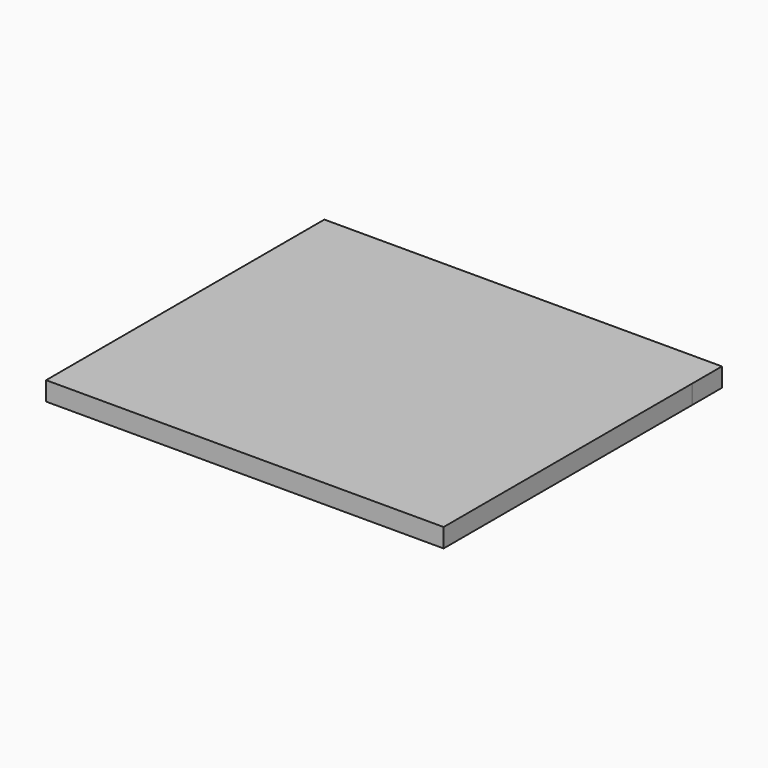
from build123d import *

# Parameters (mm, degrees)
F1_DEPTH = 19
F2_DEPTH = 548
F3_DEPTH = 548


# Not quite as in the source:
# - an extrude ends at something that could not be found from the text; its depth is read off the source's solid


with BuildPart() as f1:
    # F0 (on Top) → F1 (new body)
    with BuildSketch(Plane.XY):
        with BuildLine():
            add(Edge.make_bspline(
                [(-200, -132.6209452411), (-200, -154.8058367287), (-187.1411707237, -172.3375741418), (-168.017625666, -187.1492117643), (-133.0151869916, -187.1492117643)],
                knots=[0, 0, 0, 0, 0.4562793143, 1, 1, 1, 1], degree=3))
            Line((-200, -132.6209452411), (-200, -187.1492117643))
            Line((-200, -187.1492117643), (-133.0151869916, -187.1492117643))
        make_face()
        with BuildLine():
            Line((200, -187.1492117643), (200, -133.3316862583))
            add(Edge.make_bspline(
                [(200, -133.3316862583), (196.8726040376, -145.854416396), (194.7195639705, -177.063078406), (166.3433221251, -183.7126432901), (157.4708074331, -187.1492117643)],
                knots=[0, 0, 0, 0, 0.5227747717, 1, 1, 1, 1], degree=3))
            Line((157.4708074331, -187.1492117643), (200, -187.1492117643))
        make_face()
        with BuildLine():
            add(Edge.make_bspline(
                [(200, 125.7612258196), (200.0567834577, 125.2951155246), (200.0345329904, 125.1404634173), (200, 124.9924004078)],
                knots=[0.9249687191, 0.9249687191, 0.9249687191, 0.9249687191, 1, 1, 1, 1], degree=3))
            Line((200, 125.7612258196), (200, 124.9924004078))
        make_face()
        with BuildLine():
            add(Edge.make_bspline(
                [(159.7772687674, 162.8507882357), (169.0774328446, 160.2876502356), (193.3291623418, 156.440564551), (199.6711808851, 128.4603565342), (200, 125.7612258196)],
                knots=[0, 0, 0, 0, 0.4904809229, 0.9249687191, 0.9249687191, 0.9249687191, 0.9249687191], degree=3))
            Line((159.7772687674, 162.8507882357), (-153.6801122603, 162.8507882357))
            add(Edge.make_bspline(
                [(-200, 104.9124646716), (-200, 131.7387589341), (-185.8746875729, 148.9797410683), (-171.5849838132, 162.8507882357), (-153.6801122603, 162.8507882357)],
                knots=[0, 0, 0, 0, 0.5414752597, 1, 1, 1, 1], degree=3))
            Line((-200, 104.9124646716), (-200, -132.6209452411))
            add(Edge.make_bspline(
                [(-200, -132.6209452411), (-200, -154.8058367287), (-187.1411707237, -172.3375741418), (-168.017625666, -187.1492117643), (-133.0151869916, -187.1492117643)],
                knots=[0, 0, 0, 0, 0.4562793143, 1, 1, 1, 1], degree=3))
            Line((-133.0151869916, -187.1492117643), (157.4708074331, -187.1492117643))
            add(Edge.make_bspline(
                [(200, -133.3316862583), (196.8726040376, -145.854416396), (194.7195639705, -177.063078406), (166.3433221251, -183.7126432901), (157.4708074331, -187.1492117643)],
                knots=[0, 0, 0, 0, 0.5227747717, 1, 1, 1, 1], degree=3))
            Line((200, -133.3316862583), (200, 124.9924004078))
            Line((200, 124.9924004078), (200, 125.7612258196))
        make_face()
        with BuildLine():
            add(Edge.make_bspline(
                [(-200, 104.9124646716), (-200, 131.7387589341), (-185.8746875729, 148.9797410683), (-171.5849838132, 162.8507882357), (-153.6801122603, 162.8507882357)],
                knots=[0, 0, 0, 0, 0.5414752597, 1, 1, 1, 1], degree=3))
            Line((-153.6801122603, 162.8507882357), (-200, 162.8507882357))
            Line((-200, 162.8507882357), (-200, 104.9124646716))
        make_face()
        with BuildLine():
            Line((200, 125.7612258196), (200, 162.8507882357))
            Line((200, 162.8507882357), (159.7772687674, 162.8507882357))
            add(Edge.make_bspline(
                [(159.7772687674, 162.8507882357), (169.0774328446, 160.2876502356), (193.3291623418, 156.440564551), (199.6711808851, 128.4603565342), (200, 125.7612258196)],
                knots=[0, 0, 0, 0, 0.4904809229, 0.9249687191, 0.9249687191, 0.9249687191, 0.9249687191], degree=3))
        make_face()
    extrude(amount=F1_DEPTH)

    # F0 (on Top) → F2 (cut, through all)
    with BuildSketch(Plane.XY):
        with BuildLine():
            add(Edge.make_bspline(
                [(-200, -132.6209452411), (-200, -154.8058367287), (-187.1411707237, -172.3375741418), (-168.017625666, -187.1492117643), (-133.0151869916, -187.1492117643)],
                knots=[0, 0, 0, 0, 0.4562793143, 1, 1, 1, 1], degree=3))
            Line((-200, -132.6209452411), (-200, -187.1492117643))
            Line((-200, -187.1492117643), (-133.0151869916, -187.1492117643))
        make_face()
    extrude(amount=-F2_DEPTH, mode=Mode.SUBTRACT)

    # F0 (on Top) → F3 (cut, through all)
    with BuildSketch(Plane.XY):
        with BuildLine():
            add(Edge.make_bspline(
                [(-200, 104.9124646716), (-200, 131.7387589341), (-185.8746875729, 148.9797410683), (-171.5849838132, 162.8507882357), (-153.6801122603, 162.8507882357)],
                knots=[0, 0, 0, 0, 0.5414752597, 1, 1, 1, 1], degree=3))
            Line((-153.6801122603, 162.8507882357), (-200, 162.8507882357))
            Line((-200, 162.8507882357), (-200, 104.9124646716))
        make_face()
    extrude(amount=-F3_DEPTH, mode=Mode.SUBTRACT)


solid = f1.part
